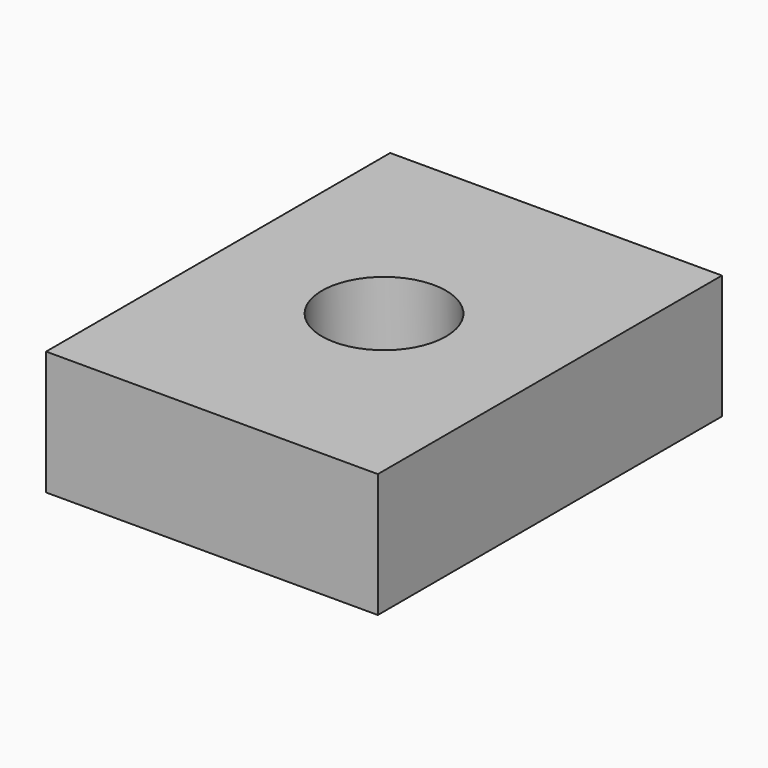
from build123d import *

# Parameters (mm, degrees)
F0_W     = 67.9279565811
F0_H     = 88.0647003651
F1_DEPTH = 25.4
F2_R     = 12.7
F3_DEPTH = 25.4


# Not quite as in the source:
# - a feature of the source that left no trace in its solid (it failed there, or was rolled back) is left out


with BuildPart() as f1:
    # F0 (on Top) → F1 (new body)
    with BuildSketch(Plane.XY):
        Rectangle(F0_W, F0_H)
    extrude(amount=F1_DEPTH)

    # F2 (on face) → F3 (cut)
    with BuildSketch(Plane.XY.offset(25.4)):
        Circle(F2_R)
    extrude(amount=-F3_DEPTH, mode=Mode.SUBTRACT)


solid = f1.part
